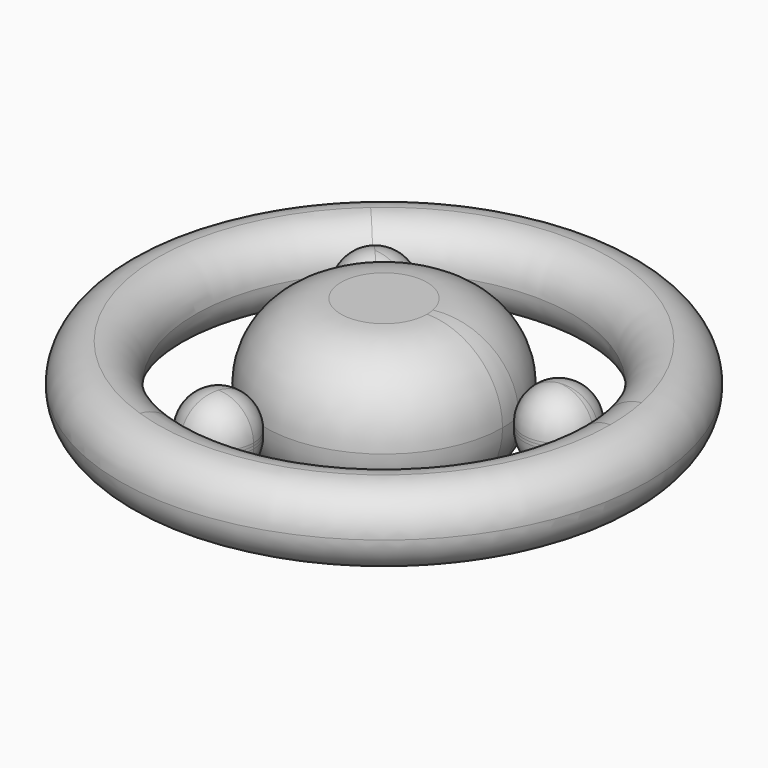
from build123d import *

# Parameters (mm, degrees)
F0_R         = 87.5
F1_DEPTH     = 12.5
F2_T4_ANGLE  = 119.9999999366
F2_T6_ANGLE  = 11.3111263795
F2_T8_ANGLE  = 108.6888739249
F2_T10_ANGLE = 119.999999759
F2_T14_ANGLE = 119.9999999366
F2_T16_ANGLE = 11.3111263795
F2_T18_ANGLE = 108.6888739249
F2_T20_ANGLE = 119.999999759
F3_DEPTH     = 12.5
F4_R         = 11.61
F4_2_R       = 11.61
F4_3_R       = 11.61
F5_DEPTH     = 25
F6_R         = 24.99999


# Not quite as in the source:
# - a fillet or chamfer that OpenCascade refuses, or shapes differently, is made with other operations: its cross-section is extruded or revolved along the edge and cut away or added
# - a fillet or chamfer is up to 0.001 mm smaller than in the source, because OpenCascade refuses the exact size


with BuildPart() as f1:
    # F0 (on Top) → F1 (new body, symmetric)
    with BuildSketch(Plane.XY):
        Circle(F0_R)
        with BuildLine():
            ThreePointArc((61.2860368058, 12.2585355016), (62.1957687482, 6.1592491279), (62.5, 0))
            ThreePointArc((62.5, 0), (36.4319504522, -50.7834912766), (-20.0268155599, -59.2045324154))
            ThreePointArc((-20.0268155599, -59.2045324154), (-61.2860368451, -12.2585353049), (-41.2592215085, 46.9459970659))
            ThreePointArc((-41.2592215085, 46.9459970659), (20.0268152781, 59.2045325108), (61.2860368058, 12.2585355016))
        make_face(mode=Mode.SUBTRACT)
    extrude(amount=F1_DEPTH, both=True)

    # F2: fillet of radius 12.5 on 10 edges, made by hand

    # F2_s1 → F2_t2 (revolve, cut)
    with BuildSketch(Plane.XZ):
        with BuildLine():
            ThreePointArc((87.5, 0), (83.8388347648, 8.8388347648), (75, 12.5))
            Line((75, 12.5), (87.5, 12.5))
            Line((87.5, 12.5), (87.5, 0))
        make_face()
    revolve(axis=Axis((0, 0, 12.5), (0, 0, 1)), mode=Mode.SUBTRACT)

    # F2_s3 → F2_t4 (revolve, cut)
    with BuildSketch(Plane(origin=(0, 0, 0), x_dir=(0, 0, 1), z_dir=(-0.7511359531, -0.6601475441, 0))):
        with BuildLine():
            ThreePointArc((12.5, 75), (8.8388347648, 66.1611652352), (0, 62.5))
            Line((0, 62.5), (12.5, 62.5))
            Line((12.5, 62.5), (12.5, 75))
        make_face()
    revolve(axis=Axis((0, 0, 12.5), (0, 0, -1)), revolution_arc=F2_T4_ANGLE, mode=Mode.SUBTRACT)

    # F2_s5 → F2_t6 (revolve, cut)
    with BuildSketch(Plane(origin=(0, 0, 0), x_dir=(0, 0, 1), z_dir=(-0.196136568, 0.9805765889, 0))):
        with BuildLine():
            ThreePointArc((12.5, 75), (8.8388347648, 66.1611652352), (0, 62.5))
            Line((0, 62.5), (12.5, 62.5))
            Line((12.5, 62.5), (12.5, 75))
        make_face()
    revolve(axis=Axis((0, 0, 12.5), (0, 0, -1)), revolution_arc=F2_T6_ANGLE, mode=Mode.SUBTRACT)

    # F2_s7 → F2_t8 (revolve, cut)
    with BuildSketch(Plane.XZ):
        with BuildLine():
            ThreePointArc((75, 12.5), (66.1611652352, 8.8388347648), (62.5, 0))
            Line((62.5, 0), (62.5, 12.5))
            Line((62.5, 12.5), (75, 12.5))
        make_face()
    revolve(axis=Axis((0, 0, 12.5), (0, 0, -1)), revolution_arc=F2_T8_ANGLE, mode=Mode.SUBTRACT)

    # F2_s9 → F2_t10 (revolve, cut)
    with BuildSketch(Plane(origin=(0, 0, 0), x_dir=(0, 0, 1), z_dir=(0.9472725186, -0.320429049, 0))):
        with BuildLine():
            ThreePointArc((12.5, 75), (8.8388347648, 66.1611652352), (0, 62.5))
            Line((0, 62.5), (12.5, 62.5))
            Line((12.5, 62.5), (12.5, 75))
        make_face()
    revolve(axis=Axis((0, 0, 12.5), (0, 0, -1)), revolution_arc=F2_T10_ANGLE, mode=Mode.SUBTRACT)

    # F2_s11 → F2_t12 (revolve, cut)
    with BuildSketch(Plane.XZ):
        with BuildLine():
            ThreePointArc((87.5, 0), (83.8388347648, -8.8388347648), (75, -12.5))
            Line((75, -12.5), (87.5, -12.5))
            Line((87.5, -12.5), (87.5, 0))
        make_face()
    revolve(axis=Axis((0, 0, -12.5), (0, 0, 1)), mode=Mode.SUBTRACT)

    # F2_s13 → F2_t14 (revolve, cut)
    with BuildSketch(Plane(origin=(0, 0, 0), x_dir=(0, 0, 1), z_dir=(-0.7511359531, -0.6601475441, 0))):
        with BuildLine():
            ThreePointArc((0, 62.5), (-8.8388347648, 66.1611652352), (-12.5, 75))
            Line((-12.5, 75), (-12.5, 62.5))
            Line((-12.5, 62.5), (0, 62.5))
        make_face()
    revolve(axis=Axis((0, 0, -12.5), (0, 0, -1)), revolution_arc=F2_T14_ANGLE, mode=Mode.SUBTRACT)

    # F2_s15 → F2_t16 (revolve, cut)
    with BuildSketch(Plane(origin=(0, 0, 0), x_dir=(0, 0, 1), z_dir=(-0.196136568, 0.9805765889, 0))):
        with BuildLine():
            ThreePointArc((0, 62.5), (-8.8388347648, 66.1611652352), (-12.5, 75))
            Line((-12.5, 75), (-12.5, 62.5))
            Line((-12.5, 62.5), (0, 62.5))
        make_face()
    revolve(axis=Axis((0, 0, -12.5), (0, 0, -1)), revolution_arc=F2_T16_ANGLE, mode=Mode.SUBTRACT)

    # F2_s17 → F2_t18 (revolve, cut)
    with BuildSketch(Plane.XZ):
        with BuildLine():
            ThreePointArc((62.5, 0), (66.1611652352, -8.8388347648), (75, -12.5))
            Line((75, -12.5), (62.5, -12.5))
            Line((62.5, -12.5), (62.5, 0))
        make_face()
    revolve(axis=Axis((0, 0, -12.5), (0, 0, -1)), revolution_arc=F2_T18_ANGLE, mode=Mode.SUBTRACT)

    # F2_s19 → F2_t20 (revolve, cut)
    with BuildSketch(Plane(origin=(0, 0, 0), x_dir=(0, 0, 1), z_dir=(0.9472725186, -0.320429049, 0))):
        with BuildLine():
            ThreePointArc((0, 62.5), (-8.8388347648, 66.1611652352), (-12.5, 75))
            Line((-12.5, 75), (-12.5, 62.5))
            Line((-12.5, 62.5), (0, 62.5))
        make_face()
    revolve(axis=Axis((0, 0, -12.5), (0, 0, -1)), revolution_arc=F2_T20_ANGLE, mode=Mode.SUBTRACT)


with BuildPart() as f3:
    # F0 (on Top) → F3 (new body, symmetric)
    with BuildSketch(Plane.XY):
        with BuildLine():
            ThreePointArc((-21.9765958464, 38.221547489), (-28.8036520844, 48.8037929128), (-41.2592215085, 46.9459970659))
            ThreePointArc((-41.2592215085, 46.9459970659), (-42.3160528339, 30.5539292627), (-25.923985056, 29.4970975451))
            ThreePointArc((-25.923985056, 29.4970975451), (-23.0093577642, 33.4335962467), (-21.9765958464, 38.221547489))
        make_face()
    extrude(amount=F3_DEPTH, both=True)

    # F4
    f4_edges = [f3.edges().sort_by_distance(p)[0] for p in [
        (-28.803652, 48.803793, 12.5),
        (-42.316053, 30.553929, 12.5),
        (-23.009358, 33.433596, 12.5),
        (-28.803652, 48.803793, -12.5),
        (-42.316053, 30.553929, -12.5),
        (-23.009358, 33.433596, -12.5),
    ]]
    fillet(f4_edges, radius=F4_R)


with BuildPart() as f3b:
    # F0 (on Top) → F3, piece 2 (new body, symmetric)
    with BuildSketch(Plane.XY):
        with BuildLine():
            ThreePointArc((61.5116398612, 9.980407871), (61.4551014915, 11.1250434287), (61.2860368058, 12.2585355016))
            ThreePointArc((61.2860368058, 12.2585355016), (47.618504612, 21.3698119643), (38.5072286192, 7.7022794573))
            ThreePointArc((38.5072286192, 7.7022794573), (51.0412685892, -1.5780609469), (61.5116398612, 9.980407871))
        make_face()
    extrude(amount=F3_DEPTH, both=True)

    # F4#2
    f4_2_edges = [f3b.edges().sort_by_distance(p)[0] for p in [
        (61.455101, 11.125043, 12.5),
        (47.618505, 21.369812, 12.5),
        (51.041269, -1.578061, 12.5),
        (61.455101, 11.125043, -12.5),
        (47.618505, 21.369812, -12.5),
        (51.041269, -1.578061, -12.5),
    ]]
    fillet(f4_2_edges, radius=F4_2_R)


with BuildPart() as f3c:
    # F0 (on Top) → F3, piece 3 (new body, symmetric)
    with BuildSketch(Plane.XY):
        with BuildLine():
            ThreePointArc((-12.5832438311, -37.1993782133), (-27.3076066617, -44.4801694956), (-20.0268155599, -59.2045324154))
            ThreePointArc((-20.0268155599, -59.2045324154), (-9.5345117958, -57.6395653372), (-4.6900223335, -48.20195536))
            ThreePointArc((-4.6900223335, -48.20195536), (-6.8674196664, -41.4314374795), (-12.5832438311, -37.1993782133))
        make_face()
    extrude(amount=F3_DEPTH, both=True)

    # F4#3
    f4_3_edges = [f3c.edges().sort_by_distance(p)[0] for p in [
        (-6.86742, -41.431437, 12.5),
        (-27.307607, -44.480169, 12.5),
        (-9.534512, -57.639565, 12.5),
        (-6.86742, -41.431437, -12.5),
        (-27.307607, -44.480169, -12.5),
        (-9.534512, -57.639565, -12.5),
    ]]
    fillet(f4_3_edges, radius=F4_3_R)


with BuildPart() as f5:
    # F0 (on Top) → F5 (new body, symmetric)
    with BuildSketch(Plane.XY):
        with BuildLine():
            ThreePointArc((39.2699855458, 0), (39.0788310729, 3.8699776152), (38.5072286192, 7.7022794573))
            ThreePointArc((38.5072286192, 7.7022794573), (12.5832439583, 37.1993781703), (-25.923985056, 29.4970975451))
            ThreePointArc((-25.923985056, 29.4970975451), (-38.5072283966, -7.70228057), (-12.5832438311, -37.1993782133))
            ThreePointArc((-12.5832438311, -37.1993782133), (22.890914807, -31.9082714052), (39.2699855458, 0))
        make_face()
    extrude(amount=F5_DEPTH, both=True)

    # F6 (radius 25 in the source; OpenCascade refuses exactly that, so slightly less here)
    f6_edges = [f5.edges().sort_by_distance(p)[0] for p in [
        (39.078831, 3.869978, 25),
        (12.583244, 37.199378, 25),
        (-38.507228, -7.702281, 25),
        (22.890915, -31.908271, 25),
        (39.078831, 3.869978, -25),
        (12.583244, 37.199378, -25),
        (-38.507228, -7.702281, -25),
        (22.890915, -31.908271, -25),
    ]]
    fillet(f6_edges, radius=F6_R)


solid = Compound([f1.part, f3.part, f3b.part, f3c.part, f5.part])
